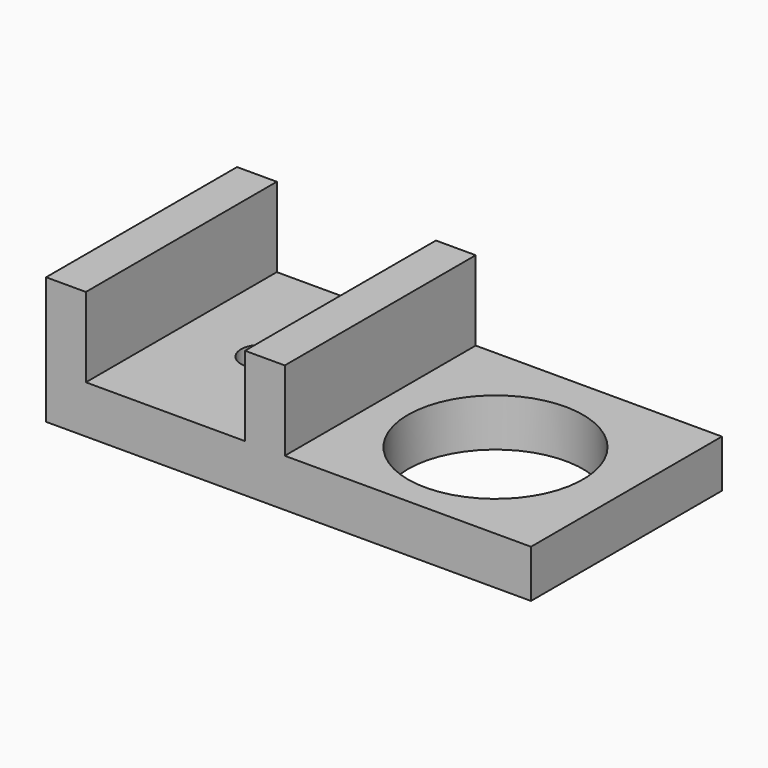
from build123d import *

# Parameters (mm, degrees)
F0_W     = 5
F0_H     = 10
F1_DEPTH = 30
F3_D     = 22
F5_D     = 5


# Not quite as in the source:
# - a feature names something its author has since deleted; it is built from what else it names


with BuildPart() as f1:
    # F0 (on Front) → F1 (new body)
    with BuildSketch(Plane.XZ):
        with Locations((-33.2201862009, 15.0932593657)):
            Rectangle(F0_W, F0_H)
        Polygon((-30.7201862009, 10.0932593657), (-35.7201862009, 10.0932593657), (-35.7201862009, 4.0932593657), (25.2284052642, 4.0932593657), (25.2284052642, 10.0932593657), (-5.7201862009, 10.0932593657), (-10.7201862009, 10.0932593657), align=None)
        with Locations((-8.2201862009, 15.0932593657)):
            Rectangle(F0_W, F0_H)
    extrude(amount=F1_DEPTH)

    # F3 (through all)
    with Locations(Plane.XY.offset(10.0932593657)):
        with Locations((9.2798137991, -15.640585908)):
            Hole(F3_D / 2)

    # F5 (through all)
    with Locations(Plane.XY.offset(10.0932593657)):
        with Locations((-20.7201862009, -15)):
            Hole(F5_D / 2)


solid = f1.part
